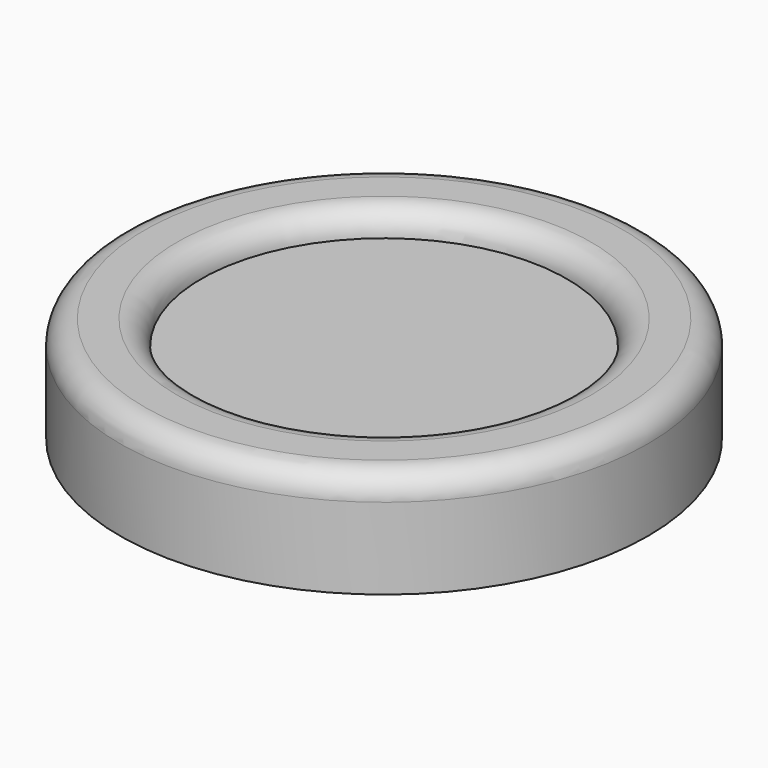
from build123d import *

# Parameters (mm, degrees)
F0_R     = 32.5
F0_R_2   = 22.5
F1_DEPTH = 10
F2_DEPTH = 13
F3_DEPTH = 8
F4_R     = 2.99999


# Not quite as in the source:
# - a fillet or chamfer is up to 0.001 mm smaller than in the source, because OpenCascade refuses the exact size


with BuildPart() as f1:
    # F0 (on Top) → F1 (new body)
    with BuildSketch(Plane.XY):
        Circle(F0_R)
        Circle(F0_R_2, mode=Mode.SUBTRACT)
        Circle(F0_R_2)
        Polygon((-8.5, 4.9074772881), (0, 9.8149545762), (8.5, 4.9074772881), (8.5, -4.9074772881), (0, -9.8149545762), (-8.5, -4.9074772881), align=None, mode=Mode.SUBTRACT)
        Polygon((8.5, 4.9074772881), (0, 9.8149545762), (-8.5, 4.9074772881), (-8.5, -4.9074772881), (0, -9.8149545762), (8.5, -4.9074772881), align=None)
    extrude(amount=F1_DEPTH)

    # F0 (on Top) → F2 (join)
    with BuildSketch(Plane.XY):
        Circle(F0_R)
        Circle(F0_R_2, mode=Mode.SUBTRACT)
    extrude(amount=F2_DEPTH)

    # F0 (on Top) → F3 (cut)
    with BuildSketch(Plane.XY):
        Polygon((8.5, 4.9074772881), (0, 9.8149545762), (-8.5, 4.9074772881), (-8.5, -4.9074772881), (0, -9.8149545762), (8.5, -4.9074772881), align=None)
    extrude(amount=F3_DEPTH, mode=Mode.SUBTRACT)

    # F4 (radius 3 in the source; OpenCascade refuses exactly that, so slightly less here)
    f4_edges = [f1.edges().sort_by_distance(p)[0] for p in [
        (-32.5, 0, 13),
        (-22.5, 0, 13),
    ]]
    fillet(f4_edges, radius=F4_R)


solid = f1.part
